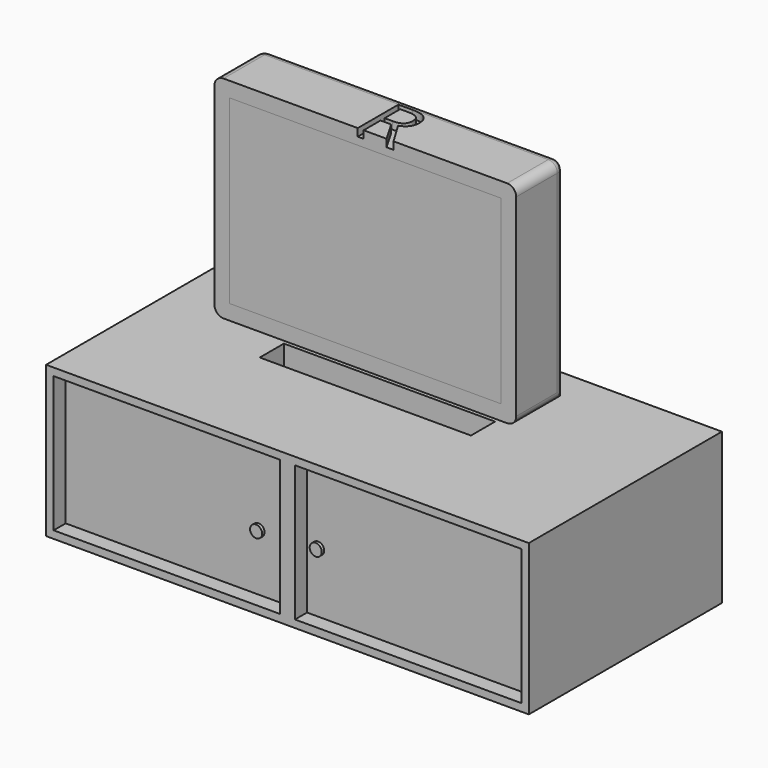
from build123d import *

# Parameters (mm, degrees)
F0_W          = 254
F0_H          = 177.8
F1_DEPTH      = 50.8
F2_T          = -12.7
F5_W          = 406.4
F5_H          = 203.2
F5_W_2        = 177.8
F5_H_2        = 25.4
F6_DEPTH      = 127
F8_W          = 190.5
F8_H          = 114.3
F9_DEPTH      = 12.7
F11_TEXT_SIZE = 190.7085875176
F12_DEPTH     = 6.35
F10_R         = 5.08
F13_DEPTH     = 2.54
F14_R         = 7.62
F15_W         = 228.6
F15_H         = 152.4
F16_DEPTH     = 25.4
F17_TEXT_SIZE = 59.9722222222
F18_DEPTH     = 6.35


# Not quite as in the source:
# - Text() gives the source's letters only with a copy of the font that has no kerning and outlines rounded to 1/6400 em; it was checked with that copy


with BuildPart() as f1:
    # F0 (on Front) → F1 (new body)
    with BuildSketch(Plane.XZ):
        with Locations((-19.5620581508, 40.2245108907)):
            Rectangle(F0_W, F0_H)
    extrude(amount=F1_DEPTH)

    # F2
    f2_openings = [f1.faces().sort_by_distance(p)[0] for p in [
        (-19.562058, -50.8, 40.224511),
    ]]
    offset(amount=F2_T, openings=f2_openings)

    # F11 (on face) → F12 (cut)
    with BuildSketch(Plane(origin=(0, 0, 0), x_dir=(-1, 0, 0), z_dir=(0, 1, 0))):
        with Locations((-43.9379418492, -28.3554891093)):
            Text('R', F11_TEXT_SIZE, font='Open Sans', text_align=(TextAlign.LEFT, TextAlign.BOTTOM))
    extrude(amount=-F12_DEPTH, mode=Mode.SUBTRACT)

    # F14
    f14_edges = [f1.edges().sort_by_distance(p)[0] for p in [
        (107.437942, -25.4, 129.124511),
        (107.437942, 0, 40.224511),
        (-19.562058, 0, 129.124511),
        (-146.562058, -25.4, 129.124511),
        (-146.562058, 0, 40.224511),
        (107.437942, -25.4, -48.675489),
        (-146.562058, -25.4, -48.675489),
    ]]
    fillet(f14_edges, radius=F14_R)

    # F17 (on face) → F18 (cut)
    with BuildSketch(Plane.XY.offset(129.1245108907)):
        with Locations((-31.8810581508, -50.8)):
            Text('R', F17_TEXT_SIZE, font='Open Sans', text_align=(TextAlign.LEFT, TextAlign.BOTTOM))
    extrude(amount=-F18_DEPTH, mode=Mode.SUBTRACT)


with BuildPart() as f6:
    # F5 (on face) → F6 (new body)
    with BuildSketch(Plane.XY.offset(-67.7254891093)):
        with Locations((-8.5096483707, -44.9975493193)):
            Rectangle(F5_W, F5_H)
        with Locations((-19.5620581508, -38.1)):
            Rectangle(F5_W_2, F5_H_2, mode=Mode.SUBTRACT)
    extrude(amount=-F6_DEPTH)

    # F8 (on face) → F9 (cut)
    with BuildSketch(Plane.XZ.offset(146.5975493193)):
        with Locations((-110.1096483707, -131.2254891093)):
            Rectangle(F8_W, F8_H)
        with Locations((93.0903516293, -131.2254891093)):
            Rectangle(F8_W, F8_H)
    extrude(amount=-F9_DEPTH, mode=Mode.SUBTRACT)


with BuildPart() as f13:
    # F10 (on face) → F13 (new body)
    with BuildSketch(Plane.XZ.offset(146.5975493193)):
        with Locations((-32.8788124025, -132.0420503616)):
            Circle(F10_R)
    extrude(amount=F13_DEPTH)


with BuildPart() as f13b:
    # F10 (on face) → F13, piece 2 (new body)
    with BuildSketch(Plane.XZ.offset(146.5975493193)):
        with Locations((17.3053424805, -129.3155252934)):
            Circle(F10_R)
    extrude(amount=F13_DEPTH)


with BuildPart() as f16:
    # F15 (on face) → F16 (new body)
    with BuildSketch(Plane.XZ.offset(50.8)):
        with Locations((-19.5620581508, 40.2245108907)):
            Rectangle(F15_W, F15_H)
    extrude(amount=-F16_DEPTH)


solid = Compound([f1.part, f6.part, f13.part, f13b.part, f16.part])
